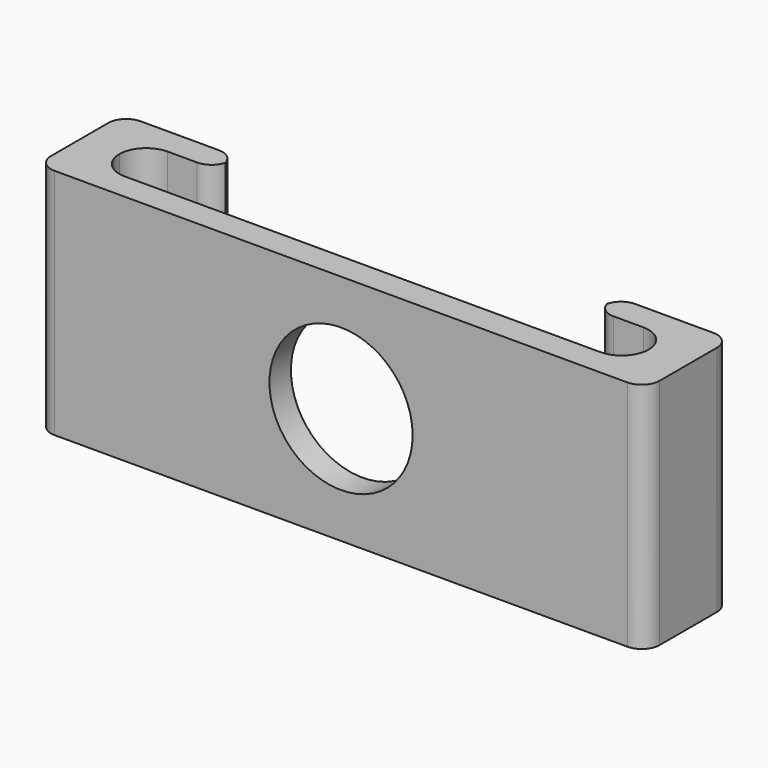
from build123d import *

# Parameters (mm, degrees)
F0_R        = 8
F1_DEPTH    = 12
F3_DEPTH    = 40
F4_T1_DEPTH = 36


# Not quite as in the source:
# - a fillet or chamfer that OpenCascade refuses, or shapes differently, is made with other operations: its cross-section is extruded or revolved along the edge and cut away or added
# - a feature names something its author has since deleted; it is built from what else it names


with BuildPart() as f1:
    # F0 (on Front) → F1 (new body)
    with BuildSketch(Plane.XZ):
        Polygon((34, 13), (-34, 13), (-34, 0), (-34, -13), (34, -13), align=None)
        Circle(F0_R, mode=Mode.SUBTRACT)
    extrude(amount=F1_DEPTH)

    # F2 (on face) → F3 (cut)
    with BuildSketch(Plane.XY.offset(13)):
        with BuildLine():
            Line((-21.2670322508, -3), (-26.5711637536, -3))
            ThreePointArc((-26.5711637536, -3), (-28.6924840972, -3.8786796564), (-29.5711637536, -6))
            ThreePointArc((-29.5711637536, -6), (-28.6924840972, -8.1213203436), (-26.5711637536, -9))
            Line((-26.5711637536, -9), (26.5711637536, -9))
            ThreePointArc((26.5711637536, -9), (28.6924840972, -8.1213203436), (29.5711637536, -6))
            ThreePointArc((29.5711637536, -6), (28.6924840972, -3.8786796564), (26.5711637536, -3))
            Line((26.5711637536, -3), (21.2670322508, -3))
            Line((21.2670322508, -3), (21.2670322508, 0))
            Line((21.2670322508, 0), (0, 0))
            Line((0, 0), (-21.2670322508, 0))
            Line((-21.2670322508, 0), (-21.2670322508, -3))
        make_face()
    extrude(amount=-F3_DEPTH, mode=Mode.SUBTRACT)

    # F4: fillet of radius 2 on 8 edges, made by hand

    # F4_s2 → F4_t1 (cut)
    with BuildSketch(Plane.XY.offset(-18)):
        with BuildLine():
            ThreePointArc((32, -12), (33.4142135624, -11.4142135624), (34, -10))
            Line((34, -10), (34, -12))
            Line((34, -12), (32, -12))
        make_face()
        with BuildLine():
            ThreePointArc((32, 0), (33.4142135624, -0.5857864376), (34, -2))
            Line((34, -2), (34, 0))
            Line((34, 0), (32, 0))
        make_face()
        with BuildLine():
            ThreePointArc((-21.2670322508, -2), (-21.8528186884, -0.5857864376), (-23.2670322508, 0))
            Line((-23.2670322508, 0), (-21.2670322508, 0))
            Line((-21.2670322508, 0), (-21.2670322508, -2))
        make_face()
        with BuildLine():
            ThreePointArc((23.2670322508, 0), (21.8528186884, -0.5857864376), (21.2670322508, -2))
            Line((21.2670322508, -2), (21.2670322508, 0))
            Line((21.2670322508, 0), (23.2670322508, 0))
        make_face()
        with BuildLine():
            ThreePointArc((-32, 0), (-33.4142135624, -0.5857864376), (-34, -2))
            Line((-34, -2), (-34, 0))
            Line((-34, 0), (-32, 0))
        make_face()
        with BuildLine():
            ThreePointArc((-34, -10), (-33.4142135624, -11.4142135624), (-32, -12))
            Line((-32, -12), (-34, -12))
            Line((-34, -12), (-34, -10))
        make_face()
        with BuildLine():
            ThreePointArc((-23.2670322508, -3), (-21.8528186884, -2.4142135624), (-21.2670322508, -1))
            Line((-21.2670322508, -1), (-21.2670322508, -3))
            Line((-21.2670322508, -3), (-23.2670322508, -3))
        make_face()
        with BuildLine():
            ThreePointArc((21.2670322508, -1), (21.8528186884, -2.4142135624), (23.2670322508, -3))
            Line((23.2670322508, -3), (21.2670322508, -3))
            Line((21.2670322508, -3), (21.2670322508, -1))
        make_face()
    extrude(amount=F4_T1_DEPTH, mode=Mode.SUBTRACT)


solid = f1.part
